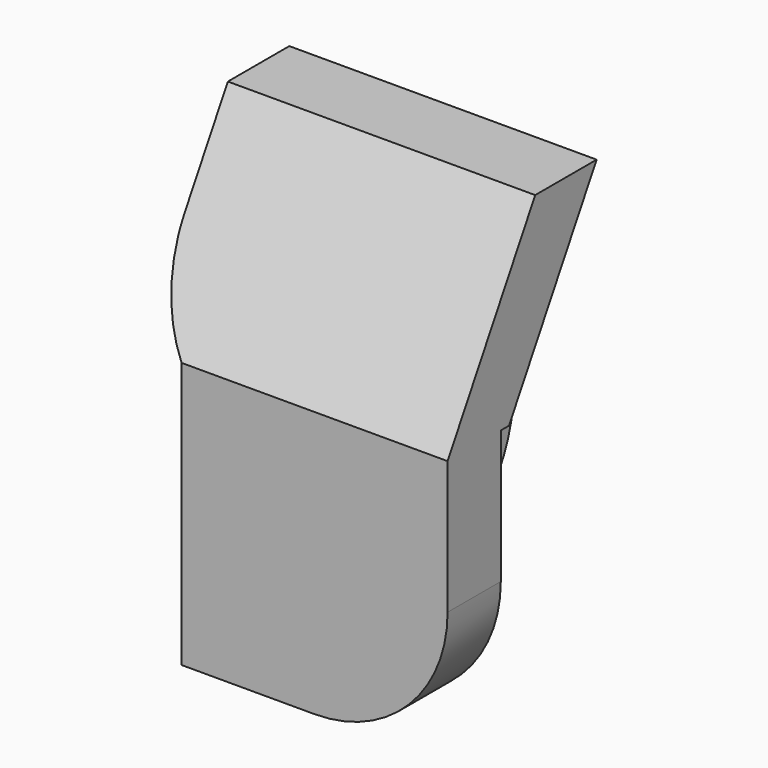
from build123d import *

# Parameters (mm, degrees)
F1_DEPTH    = 10
F4_DEPTH    = 11.5542393178
F5_D        = 3.3
F6_T1_DEPTH = 27.5
F6_T3_DEPTH = 27.5
F6_T5_DEPTH = 21.0021683442


# Not quite as in the source:
# - a fillet or chamfer that OpenCascade refuses, or shapes differently, is made with other operations: its cross-section is extruded or revolved along the edge and cut away or added


with BuildPart() as f1:
    # F0 (on Top) → F1 (new body)
    with BuildSketch(Plane.XY):
        Polygon((4.0542393178, 8.6797312124), (4.0542393178, 18.6797312124), (1.5542393178, 18.6797312124), (1.5542393178, 8.6797312124), (1.5542393178, 6.1797312124), (11.5542393178, 6.1797312124), (11.5542393178, 8.6797312124), align=None)
    extrude(amount=F1_DEPTH)

    # F3 (on Right) → F4 (join, through all)
    with BuildSketch(Plane.YZ):
        Polygon((10.296677351, 17.1307598841), (6.1797312124, 10), (9.0664825583, 10), (13.183428697, 17.1307598841), align=None)
    extrude(amount=F4_DEPTH)

    # F5 (through all)
    with Locations(Plane.YZ.offset(4.0542393178)):
        with Locations((11.6797312124, 5)):
            Hole(F5_D / 2)

    # F6: fillet of radius 5 on 4 edges, made by hand

    # F6_s2 → F6_t1 (cut)
    with BuildSketch(Plane.YZ.offset(-10.9457606822)):
        with BuildLine():
            ThreePointArc((13.6797312124, 0), (17.2152651183, 1.4644660941), (18.6797312124, 5))
            Line((18.6797312124, 5), (18.6797312124, 0))
            Line((18.6797312124, 0), (13.6797312124, 0))
        make_face()
        with BuildLine():
            ThreePointArc((18.6797312124, 5), (17.2152651183, 8.5355339059), (13.6797312124, 10))
            Line((13.6797312124, 10), (18.6797312124, 10))
            Line((18.6797312124, 10), (18.6797312124, 5))
        make_face()
    extrude(amount=F6_T1_DEPTH, mode=Mode.SUBTRACT)

    # F6_s4 → F6_t3 (cut)
    with BuildSketch(Plane.XZ.offset(-21.1797312124)):
        with BuildLine():
            ThreePointArc((6.5542393178, 0), (10.0897732237, 1.4644660941), (11.5542393178, 5))
            Line((11.5542393178, 5), (11.5542393178, 0))
            Line((11.5542393178, 0), (6.5542393178, 0))
        make_face()
    extrude(amount=F6_T3_DEPTH, mode=Mode.SUBTRACT)

    # F6_s6 → F6_t5 (cut)
    with BuildSketch(Plane.XZ.offset(-18.1241910575)):
        with BuildLine():
            ThreePointArc((1.5542393178, 10), (0.4049590094, 11.6518912998), (0, 13.6230833997))
            Line((0, 13.6230833997), (0, 10))
            Line((0, 10), (1.5542393178, 10))
        make_face()
    extrude(amount=F6_T5_DEPTH, mode=Mode.SUBTRACT)


solid = f1.part
